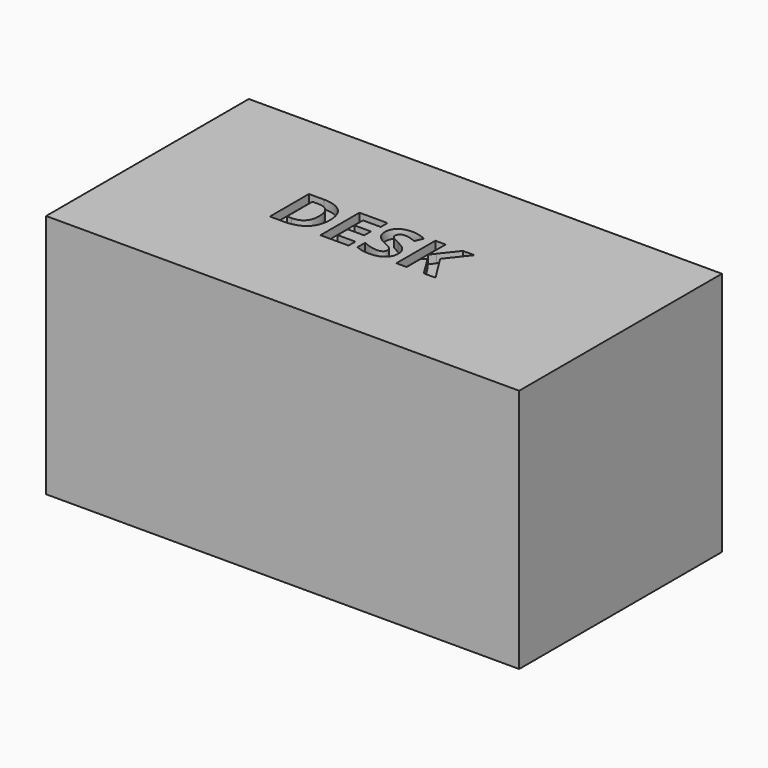
from build123d import *

# Parameters (mm, degrees)
F0_W         = 1422.4
F0_H         = 762
F1_DEPTH     = 736.6
F2_TEXT_SIZE = 205.3822080294
F3_DEPTH     = 25.4


# Not quite as in the source:
# - Text() gives the source's letters only with a copy of the font that has no kerning and outlines rounded to 1/6400 em; it was checked with that copy


with BuildPart() as f1:
    # F0 (on Top) → F1 (new body)
    with BuildSketch(Plane.XY):
        with Locations((711.2, 381)):
            Rectangle(F0_W, F0_H)
    extrude(amount=F1_DEPTH)

    # F2 (on face) → F3 (cut)
    with BuildSketch(Plane.XY.offset(736.6)):
        with Locations((393.4701383114, 326.1545300484)):
            Text('DESK', F2_TEXT_SIZE, font='Open Sans', font_style=FontStyle.BOLD, text_align=(TextAlign.LEFT, TextAlign.BOTTOM))
    extrude(amount=-F3_DEPTH, mode=Mode.SUBTRACT)


solid = f1.part
